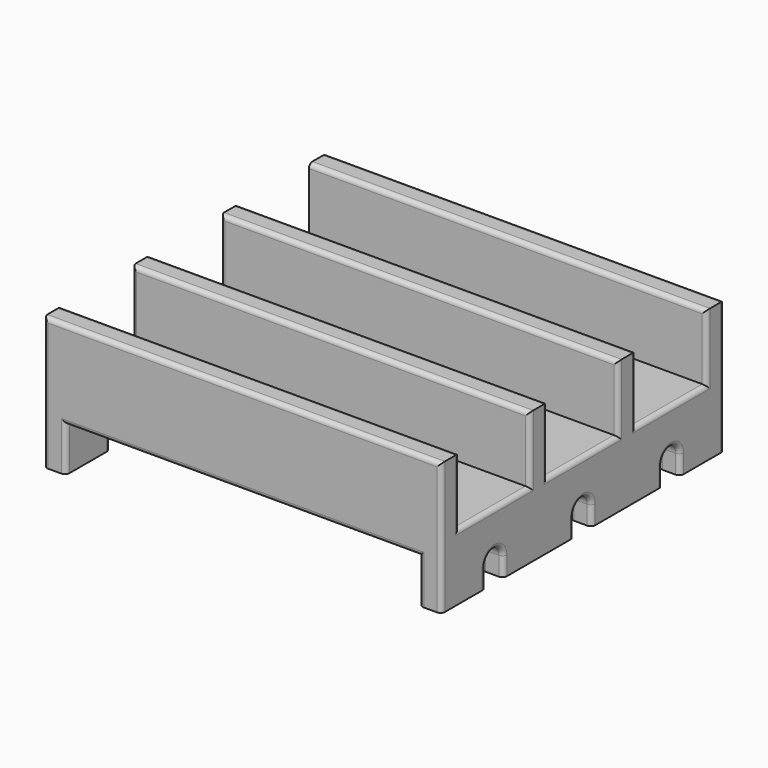
from build123d import *

# Parameters (mm, degrees)
F1_DEPTH = 90
F3_DEPTH = 90
F4_W     = 20
F4_H     = 30
F5_DEPTH = 90
F6_W     = 80
F6_H     = 10
F7_DEPTH = 90
F8_R     = 1


with BuildPart() as f1:
    # F0 (on Right) → F1 (new body)
    with BuildSketch(Plane.YZ):
        Polygon((-2.5, 30), (-2.5, 0), (0, 0), (77.5, 0), (77.5, 30), align=None)
    extrude(amount=F1_DEPTH)

    # F2 (on Right) → F3 (cut)
    with BuildSketch(Plane.YZ):
        with BuildLine():
            ThreePointArc((10, 4.2626853101), (12.5, 1.7626853101), (15, 4.2626853101))
            ThreePointArc((15, 4.2626853101), (12.5, 6.7626853101), (10, 4.2626853101))
        make_face()
        with BuildLine():
            Line((15, 0), (15, 4.2626853101))
            ThreePointArc((15, 4.2626853101), (12.5, 1.7626853101), (10, 4.2626853101))
            Line((10, 4.2626853101), (10, 0))
            Line((10, 0), (15, 0))
        make_face()
        with BuildLine():
            ThreePointArc((35, 4.2626853101), (37.5, 1.7626853101), (40, 4.2626853101))
            ThreePointArc((40, 4.2626853101), (37.5, 6.7626853101), (35, 4.2626853101))
        make_face()
        with BuildLine():
            Line((40, 0), (40, 4.2626853101))
            ThreePointArc((40, 4.2626853101), (37.5, 1.7626853101), (35, 4.2626853101))
            Line((35, 4.2626853101), (35, 0))
            Line((35, 0), (40, 0))
        make_face()
        with BuildLine():
            ThreePointArc((60, 4.2626853101), (62.5, 1.7626853101), (65, 4.2626853101))
            ThreePointArc((65, 4.2626853101), (62.5, 6.7626853101), (60, 4.2626853101))
        make_face()
        with BuildLine():
            Line((65, 0), (65, 4.2626853101))
            ThreePointArc((65, 4.2626853101), (62.5, 1.7626853101), (60, 4.2626853101))
            Line((60, 4.2626853101), (60, 0))
            Line((60, 0), (65, 0))
        make_face()
    extrude(amount=F3_DEPTH, mode=Mode.SUBTRACT)

    # F4 (on Right) → F5 (cut)
    with BuildSketch(Plane.YZ):
        with Locations((12.4999999974, 30)):
            Rectangle(F4_W, F4_H)
        with Locations((37.4999999974, 30)):
            Rectangle(F4_W, F4_H)
        with Locations((62.4999999974, 30)):
            Rectangle(F4_W, F4_H)
    extrude(amount=F5_DEPTH, mode=Mode.SUBTRACT)

    # F6 (on face) → F7 (cut)
    with BuildSketch(Plane.XZ.offset(2.5)):
        with Locations((45, 5)):
            Rectangle(F6_W, F6_H)
    extrude(amount=-F7_DEPTH, mode=Mode.SUBTRACT)

    # F8
    f8_edges = [f1.edges().sort_by_distance(p)[0] for p in [
        (45, -2.5, 30),
        (45, 22.5, 30),
        (45, 47.5, 30),
        (45, 72.5, 30),
        (45, 27.5, 30),
        (45, 52.5, 30),
        (90, 12.5, 15),
        (90, 37.5, 15),
        (90, 62.5, 15),
        (90, -2.5, 15),
        (0, -2.5, 15),
        (45, -2.5, 10),
        (45, 77.5, 30),
        (5, -2.5, 5),
        (85, -2.5, 5),
        (85, 15, 2.131343),
        (85, 35, 2.131343),
        (85, 60, 2.131343),
        (5, 15, 2.131343),
        (5, 35, 2.131343),
        (5, 60, 2.131343),
        (90, 77.5, 15),
        (0, 77.5, 15),
        (0, 22.5, 22.5),
        (0, 27.5, 22.5),
        (0, 47.5, 22.5),
        (0, 52.5, 22.5),
        (0, 2.5, 22.5),
        (90, 27.5, 22.5),
        (90, 22.5, 22.5),
        (90, 2.5, 22.5),
        (90, 47.5, 22.5),
        (90, 52.5, 22.5),
        (90, 72.5, 22.5),
        (45, 2.5, 30),
        (90, 15, 2.131343),
        (90, 40, 2.131343),
        (90, 65, 2.131343),
        (0, 65, 2.131343),
        (0, 40, 2.131343),
        (0, 15, 2.131343),
        (0, 12.5, 15),
        (0, 37.5, 15),
        (0, 62.5, 15),
        (0, 62.5, 6.762685),
        (0, 60, 2.131343),
        (0, 37.5, 6.762685),
        (0, 35, 2.131343),
        (0, 12.5, 6.762685),
        (0, 10, 2.131343),
        (5, 10, 2.131343),
        (5, 12.5, 6.762685),
        (5, 37.5, 6.762685),
        (5, 40, 2.131343),
        (5, 62.5, 6.762685),
        (5, 65, 2.131343),
        (45, 77.5, 10),
        (85, 65, 2.131343),
        (85, 62.5, 6.762685),
        (85, 40, 2.131343),
        (85, 37.5, 6.762685),
        (85, 12.5, 6.762685),
        (85, 10, 2.131343),
        (90, 62.5, 6.762685),
        (90, 60, 2.131343),
        (90, 37.5, 6.762685),
        (90, 35, 2.131343),
        (90, 12.5, 6.762685),
        (90, 10, 2.131343),
    ]]
    fillet(f8_edges, radius=F8_R)


solid = f1.part
